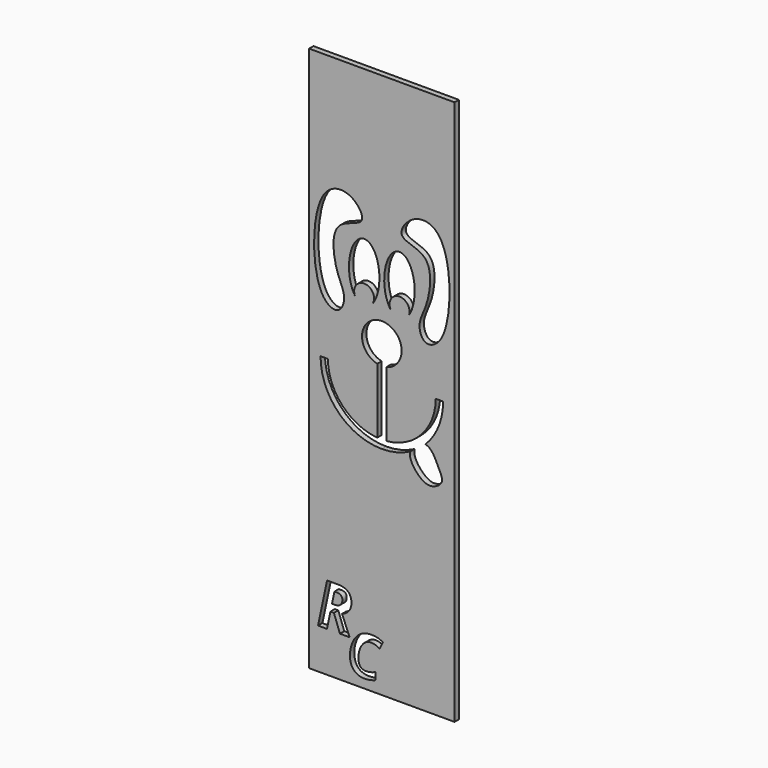
from build123d import *

# Parameters (mm, degrees)
F0_W           = 40
F0_H           = 150
F1_DEPTH       = 1.5
F3_DEPTH       = 25
F4_TEXT_SIZE   = 15.2964507126
F4_TEXT_SIZE_2 = 16.4477878975
F5_DEPTH       = 25


# Not quite as in the source:
# - ends of sketch curves that miss each other by under 0.0002 mm in the source are joined
# - Text() gives the source's letters only with a copy of the font that has no kerning and outlines rounded to 1/6400 em; it was checked with that copy


with BuildPart() as f1:
    # F0 (on Front) → F1 (new body)
    with BuildSketch(Plane.XZ):
        with Locations((-20, -1.5640810132)):
            Rectangle(F0_W, F0_H)
    extrude(amount=F1_DEPTH)

    # F2 (on face) → F3 (cut)
    with BuildSketch(Plane.XZ.offset(1.5)):
        with BuildLine():
            ThreePointArc((-27.4219227263, 17.7540056808), (-24.7749440678, 21.488621809), (-22.3862708579, 17.5837410247))
            add(Edge.make_bspline(
                [(-22.3862708579, 17.5837410247), (-12.2475826241, 31.8853910361), (-24.7730657056, 32.3089006679), (-37.2985487871, 32.7324102998), (-27.4219227263, 17.7540056808)],
                knots=[0.6277986958, 0.6277986958, 0.6277986958, 3.1241983587, 3.1241983587, 5.6205980217, 5.6205980217, 5.6205980217], degree=2, weights=[1, 0.3170301828, 1, 0.3170301828, 1]))
        make_face()
        with BuildLine():
            add(Edge.make_bspline(
                [(-25.5937585235, 36.4895239472), (-24.8840037593, 37.759035981), (-28.1815148217, 42.8700210609), (-39.3668621474, 41.9417745088), (-39.447524575, 14.7153205258), (-31.5379321358, 11.3761128353), (-29.6133465757, 17.0370300653), (-32.9392574821, 21.7669860003), (-34.5091962772, 34.9335617144), (-26.3932706947, 35.0594661672), (-25.5937585235, 36.4895239472)],
                knots=[0, 0, 0, 0, 0.1035637264, 0.2250312209, 0.4398690484, 0.5418287869, 0.6298402252, 0.7388699663, 0.8833393392, 1, 1, 1, 1], degree=3))
        make_face()
        with BuildLine():
            ThreePointArc((-17.6137291421, 17.5837410247), (-15.2250559322, 21.488621809), (-12.5780772737, 17.7540056808))
            add(Edge.make_bspline(
                [(-12.5780772737, 17.7540056808), (-2.7014512129, 32.7324102998), (-15.2269342944, 32.3089006679), (-27.7524173759, 31.8853910361), (-17.6137291421, 17.5837410247)],
                knots=[0.6625872855, 0.6625872855, 0.6625872855, 3.1589869485, 3.1589869485, 5.6553866114, 5.6553866114, 5.6553866114], degree=2, weights=[1, 0.3170301828, 1, 0.3170301828, 1]))
        make_face()
        with BuildLine():
            add(Edge.make_bspline(
                [(-14.4062414765, 36.4895239472), (-15.1159962407, 37.759035981), (-11.8184851783, 42.8700210609), (-0.6331378526, 41.9417745088), (-0.552475425, 14.7153205258), (-8.4620678642, 11.3761128353), (-10.3866534243, 17.0370300653), (-7.0607425179, 21.7669860003), (-5.4908037228, 34.9335617144), (-13.6067293053, 35.0594661672), (-14.4062414765, 36.4895239472)],
                knots=[0, 0, 0, 0, 0.1035637264, 0.2250312209, 0.4398690484, 0.5418287869, 0.6298402252, 0.7388699663, 0.8833393392, 1, 1, 1, 1], degree=3))
        make_face()
        with BuildLine():
            Line((-20, 3.0913549211), (-20, 13.9789943848))
            ThreePointArc((-20, 13.9789943848), (-25.4073338175, 9.1643918323), (-21.25, 3.236809502))
            ThreePointArc((-21.25, 3.236809502), (-20.6292171793, 3.1278408354), (-20, 3.0913549211))
        make_face()
        with BuildLine():
            ThreePointArc((-14.5561802681, 8.5351746529), (-16.150638152, 12.3845365009), (-20, 13.9789943848))
            Line((-20, 13.9789943848), (-20, 3.0913549211))
            ThreePointArc((-20, 3.0913549211), (-19.3707828207, 3.1278408354), (-18.75, 3.236809502))
            ThreePointArc((-18.75, 3.236809502), (-15.7315138551, 5.1565359768), (-14.5561802681, 8.5351746529))
        make_face()
        with BuildLine():
            Line((-20, -14.7056328334), (-20, 3.0913549211))
            ThreePointArc((-20, 3.0913549211), (-20.6292171793, 3.1278408354), (-21.25, 3.236809502))
            Line((-21.25, 3.236809502), (-21.25, -14.6529477252))
            ThreePointArc((-21.25, -14.6529477252), (-20.6255554418, -14.6924686178), (-20, -14.7056328334))
        make_face()
        with BuildLine():
            ThreePointArc((-18.75, 3.236809502), (-19.3707828207, 3.1278408354), (-20, 3.0913549211))
            Line((-20, 3.0913549211), (-20, -14.7056328334))
            ThreePointArc((-20, -14.7056328334), (-19.3744478244, -14.6924170637), (-18.7500086967, -14.6528448922))
            Line((-18.7500086967, -14.6528448922), (-18.75, 3.236809502))
        make_face()
        with BuildLine():
            ThreePointArc((-18.7500086967, -14.6528448922), (-19.3744478244, -14.6924170637), (-20, -14.7056328334))
            Line((-20, -14.7056328334), (-20, -16.9841182179))
            ThreePointArc((-20, -16.9841182179), (-15.9892421877, -16.4993916545), (-12.2093368196, -15.0733995511))
            add(Edge.make_bspline(
                [(-8.0176050551, -11.9761889788), (-9.6280215791, -11.7153102699), (-11.8275827109, -13.2713045816), (-12.2093368196, -15.0733995511)],
                knots=[0.8192656785, 0.8192656785, 0.8192656785, 0.8192656785, 1, 1, 1, 1], degree=3))
            ThreePointArc((-8.0176050551, -11.9761889788), (-4.3946282088, -6.4725350611), (-3.1607491398, 0))
            Line((-3.1607491398, 0), (-5.1607491398, 0))
            ThreePointArc((-5.1607491398, 0), (-9.119329802, -9.9566093232), (-18.7500086967, -14.6528448922))
        make_face()
        with BuildLine():
            Line((-20, -16.9841182179), (-20, -14.7056328334))
            ThreePointArc((-20, -14.7056328334), (-20.6255554418, -14.6924686178), (-21.25, -14.6529477252))
            ThreePointArc((-21.25, -14.6529477252), (-30.8814773614, -9.9570600979), (-34.8404760957, 0))
            Line((-34.8404760957, 0), (-36.8404760957, 0))
            ThreePointArc((-36.8404760957, 0), (-31.9590891216, -12.0009805701), (-20, -16.9841182179))
        make_face()
        with BuildLine():
            ThreePointArc((-8.0176050551, -11.9761889788), (-9.9929281233, -13.6879356242), (-12.2093368196, -15.0733995511))
            add(Edge.make_bspline(
                [(-12.2093368196, -15.0733995511), (-12.6211262563, -17.0172782301), (-9.648696883, -20.9092270341), (-6.4032408639, -22.0633598385), (-2.6506699354, -19.894698825), (-4.4852882747, -16.2240246824), (-6.359829525, -12.2447395888), (-8.0176050551, -11.9761889788)],
                knots=[0, 0, 0, 0, 0.1949539842, 0.3402123099, 0.4818034971, 0.6332163358, 0.8192656785, 0.8192656785, 0.8192656785, 0.8192656785], degree=3))
        make_face()
        with BuildLine():
            add(Edge.make_bspline(
                [(-8.0176050551, -11.9761889788), (-9.6280215791, -11.7153102699), (-11.8275827109, -13.2713045816), (-12.2093368196, -15.0733995511)],
                knots=[0.8192656785, 0.8192656785, 0.8192656785, 0.8192656785, 1, 1, 1, 1], degree=3))
            ThreePointArc((-12.2093368196, -15.0733995511), (-9.9929281233, -13.6879356242), (-8.0176050551, -11.9761889788))
        make_face()
    extrude(amount=-F3_DEPTH, mode=Mode.SUBTRACT)

    # F4 (on face) → F5 (cut)
    with BuildSketch(Plane.XZ.offset(1.5)):
        with Locations((-29.6751074493, -73.9780217409)):
            Text('C', F4_TEXT_SIZE, font='Open Sans', font_style=FontStyle.BOLDITALIC, text_align=(TextAlign.LEFT, TextAlign.BOTTOM))
        with Locations((-37.9647947848, -65.4514804482)):
            Text('R', F4_TEXT_SIZE_2, font='Open Sans', font_style=FontStyle.BOLDITALIC, text_align=(TextAlign.LEFT, TextAlign.BOTTOM))
    extrude(amount=-F5_DEPTH, mode=Mode.SUBTRACT)


solid = f1.part
